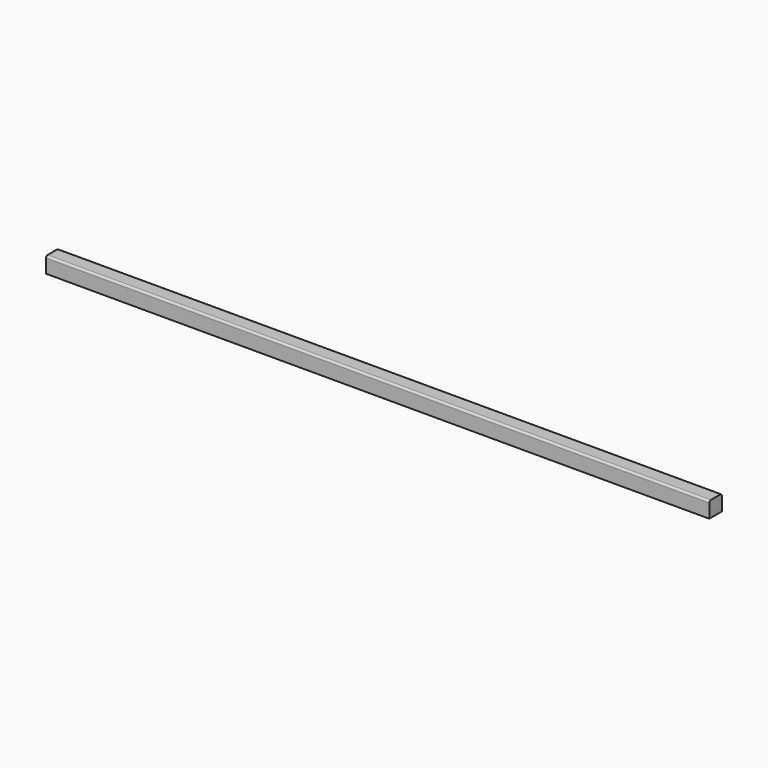
from build123d import *

# Parameters (mm, degrees)
F2_DEPTH = 533.4


# Not quite as in the source:
# - a variable given as a bare number and used for a length is read in inches; the dataset says mm whatever the document's units were


with BuildPart() as f2:
    # F1 (on Right) → F2 (new body)
    with BuildSketch(Plane.YZ):
        with BuildLine():
            Line((-6.35, -6.35), (6.35, -6.35))
            Line((6.35, -6.35), (6.35, 4.7625))
            ThreePointArc((6.35, 4.7625), (5.8850320151, 5.8850320151), (4.7625, 6.35))
            Line((4.7625, 6.35), (-4.7625, 6.35))
            ThreePointArc((-4.7625, 6.35), (-5.8850320151, 5.8850320151), (-6.35, 4.7625))
            Line((-6.35, 4.7625), (-6.35, -6.35))
        make_face()
    extrude(amount=-F2_DEPTH)


solid = f2.part
